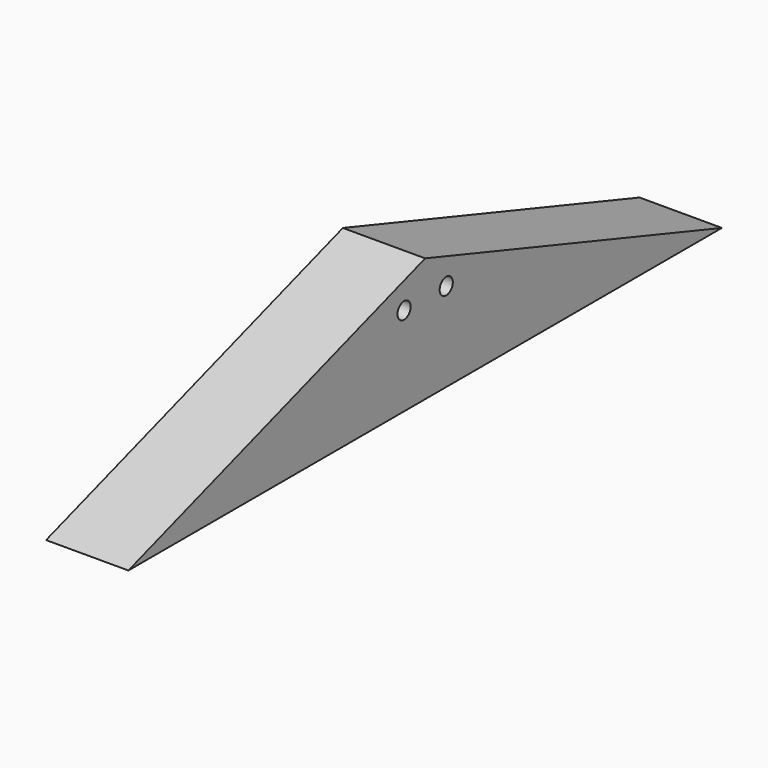
from build123d import *

# Parameters (mm, degrees)
F1_DEPTH  = 8
F3_DEPTH  = 621.7
F4_DEPTH  = 5.5
F7_DEPTH  = 5.5
F9_DEPTH  = 5.5
F11_DEPTH = 5.5
F13_DEPTH = 5.5
F15_DEPTH = 5.5
F17_DEPTH = 308.2
F18_DEPTH = 24
F20_DEPTH = 244.2
F21_DEPTH = 30.35
F22_R     = 2.5
F23_DEPTH = 0.5
F24_R     = 2.5
F25_DEPTH = 0.5
F26_R     = 2.5
F27_DEPTH = 0.5
F28_R     = 2.5
F29_DEPTH = 0.5
F30_W     = 14.1428571429
F30_H     = 18
F30_W_2   = 4.1785714286
F30_H_2   = 6.1071428571
F31_DEPTH = 0.5
F32_DEPTH = 25
F34_DEPTH = 8


# Not quite as in the source:
# - a feature of the source that left no trace in its solid (it failed there, or was rolled back) is left out


with BuildPart() as f1:
    # F0 (on Top) → F1 (new body)
    with BuildSketch(Plane.XY):
        Polygon((-327.3, 108.1424002851), (-327.3, -140.8575997149), (-102.6, -140.8575997149), (-102.6, -170.8575997149), (0, -170.8575997149), (0, -140.8575997149), (288.9, -140.8575997149), (288.9, 108.1424002851), (0, 108.1424002851), (0, 138.1424002851), (-102.6, 128.6424002851), (-102.6, 108.1424002851), align=None)
    extrude(amount=F1_DEPTH)

    # F2 (on face) → F3 (join)
    with BuildSketch(Plane.YZ.offset(288.9)):
        Polygon((-16.3575997149, 51.4532495908), (-146.3575997149, 8), (-140.8575997149, 8), (108.1424002851, 8), (113.6424002851, 8), align=None)
    extrude(amount=-F3_DEPTH)

    # F2 (on face) → F4 (join)
    with BuildSketch(Plane.YZ.offset(288.9)):
        Polygon((-16.3575997149, 51.4532495908), (-146.3575997149, 8), (113.6424002851, 8), align=None)
    extrude(amount=F4_DEPTH)

    # F5 (on face) → F7 (join)
    with BuildSketch(Plane.XZ.offset(170.8575997149)):
        Polygon((-51.3, 62.75), (-108.1, 8), (5.5, 8), align=None)
    extrude(amount=F7_DEPTH)

    # F8 (on face) → F9 (cut)
    with BuildSketch(Plane(origin=(-13.187163576, 142.4213666207, 0), x_dir=(-0.9957406741, -0.0921982106, 0), z_dir=(-0.0921982106, 0.9957406741, 0))):
        Polygon((91.8565413643, 4.3927081219), (38.2758658123, 55.8195932448), (-15.3048097397, 4.3927081219), align=None)
    extrude(amount=-F9_DEPTH, mode=Mode.SUBTRACT)

    # F10 (on face) → F11 (cut)
    with BuildSketch(Plane(origin=(-332.8, 0, 0), x_dir=(0, -1, 0), z_dir=(-1, 0, 0))):
        Polygon((144.6140170728, 2.7836871671), (16.3575997149, 45.6541342062), (-111.8988176431, 2.7836871671), align=None)
    extrude(amount=-F11_DEPTH, mode=Mode.SUBTRACT)

    # F12 (on face) → F13 (cut)
    with BuildSketch(Plane.YZ.offset(294.4)):
        Polygon((111.8988176431, 2.7836871671), (-16.3575997149, 45.6541342062), (-144.6140170728, 2.7836871671), align=None)
    extrude(amount=-F13_DEPTH, mode=Mode.SUBTRACT)

    # F14 (on face) → F15 (cut)
    with BuildSketch(Plane.XZ.offset(176.3575997149)):
        Polygon((1.6830285492, 4.0401099834), (-51.3, 55.1108989459), (-104.2830285492, 4.0401099834), align=None)
    extrude(amount=-F15_DEPTH, mode=Mode.SUBTRACT)

    # F16 (on face) → F17 (join)
    with BuildSketch(Plane.YZ.offset(294.4)):
        Polygon((-37.9123742622, 48.4659791319), (-36.6443145321, 44.6722981882), (-16.3575997149, 51.4532495908), (3.9291151024, 44.6722981882), (5.1971748325, 48.4659791319), (-16.3575997149, 55.670786811), align=None)
    extrude(amount=-F17_DEPTH)

    # F16 (on face) → F18 (cut)
    with BuildSketch(Plane.YZ.offset(294.4)):
        Polygon((-37.9123742622, 48.4659791319), (-36.6443145321, 44.6722981882), (-16.3575997149, 51.4532495908), (3.9291151024, 44.6722981882), (5.1971748325, 48.4659791319), (-16.3575997149, 55.670786811), align=None)
    extrude(amount=-F18_DEPTH, mode=Mode.SUBTRACT)

    # F19 (on face) → F20 (join)
    with BuildSketch(Plane(origin=(-332.8, 0, 0), x_dir=(0, -1, 0), z_dir=(-1, 0, 0))):
        Polygon((-5.1971748325, 48.4659791319), (-3.9291151024, 44.6722981882), (16.3575997149, 51.4532495908), (36.6443145321, 44.6722981882), (37.9123742622, 48.4659791319), (16.3575997149, 55.670786811), align=None)
    extrude(amount=-F20_DEPTH)

    # F19 (on face) → F21 (cut)
    with BuildSketch(Plane(origin=(-332.8, 0, 0), x_dir=(0, -1, 0), z_dir=(-1, 0, 0))):
        Polygon((-5.1971748325, 48.4659791319), (-3.9291151024, 44.6722981882), (16.3575997149, 51.4532495908), (36.6443145321, 44.6722981882), (37.9123742622, 48.4659791319), (16.3575997149, 55.670786811), align=None)
    extrude(amount=-F21_DEPTH, mode=Mode.SUBTRACT)

    # F22 (on face) → F23 (cut)
    with BuildSketch(Plane(origin=(-327.3, 0, 0), x_dir=(0, -1, 0), z_dir=(-1, 0, 0))):
        with Locations((8.3575997149, 35)):
            Circle(F22_R)
        with Locations((24.3575997149, 35)):
            Circle(F22_R)
    extrude(amount=-F23_DEPTH, mode=Mode.SUBTRACT)

    # F24 (on face) → F25 (cut)
    with BuildSketch(Plane.YZ.offset(288.9)):
        with Locations((-24.3575997149, 35)):
            Circle(F24_R)
        with Locations((-8.3575997149, 35)):
            Circle(F24_R)
    extrude(amount=-F25_DEPTH, mode=Mode.SUBTRACT)

    # F26 (on face) → F27 (cut)
    with BuildSketch(Plane.XZ.offset(170.8575997149)):
        with Locations((-59.3, 35)):
            Circle(F26_R)
        with Locations((-43.3, 35)):
            Circle(F26_R)
    extrude(amount=-F27_DEPTH, mode=Mode.SUBTRACT)

    # F28 (on face) → F29 (cut)
    with BuildSketch(Plane(origin=(-12.6822332802, 136.9681194259, 0), x_dir=(-0.9957406741, -0.0921982106, 0), z_dir=(-0.0921982106, 0.9957406741, 0))):
        with Locations((30.7829559704, 35)):
            Circle(F28_R)
        with Locations((46.7829559704, 35)):
            Circle(F28_R)
    extrude(amount=-F29_DEPTH, mode=Mode.SUBTRACT)

    # F30 (on face) → F31 (cut)
    with BuildSketch(Plane.YZ.offset(288.9)):
        with Locations((-16.3575997149, 14)):
            Rectangle(F30_W, F30_H)
        with Locations((-19.4111711434, 9.9821428571)):
            Rectangle(F30_W_2, F30_H_2, mode=Mode.SUBTRACT)
        with Locations((-13.3040282863, 9.9821428571)):
            Rectangle(F30_W_2, F30_H_2, mode=Mode.SUBTRACT)
        with Locations((-19.4111711434, 18.0178571429)):
            Rectangle(F30_W_2, F30_H_2, mode=Mode.SUBTRACT)
        with Locations((-13.3040282863, 18.0178571429)):
            Rectangle(F30_W_2, F30_H_2, mode=Mode.SUBTRACT)
        with Locations((18.6424002851, 14)):
            Rectangle(F30_W, F30_H)
        with Locations((15.5888288566, 9.9821428571)):
            Rectangle(F30_W_2, F30_H_2, mode=Mode.SUBTRACT)
        with Locations((21.6959717137, 9.9821428571)):
            Rectangle(F30_W_2, F30_H_2, mode=Mode.SUBTRACT)
        with Locations((15.5888288566, 18.0178571429)):
            Rectangle(F30_W_2, F30_H_2, mode=Mode.SUBTRACT)
        with Locations((21.6959717137, 18.0178571429)):
            Rectangle(F30_W_2, F30_H_2, mode=Mode.SUBTRACT)
        with Locations((-51.3575997149, 14)):
            Rectangle(F30_W, F30_H)
        with Locations((-54.4111711434, 9.9821428571)):
            Rectangle(F30_W_2, F30_H_2, mode=Mode.SUBTRACT)
        with Locations((-48.3040282863, 9.9821428571)):
            Rectangle(F30_W_2, F30_H_2, mode=Mode.SUBTRACT)
        with Locations((-54.4111711434, 18.0178571429)):
            Rectangle(F30_W_2, F30_H_2, mode=Mode.SUBTRACT)
        with Locations((-48.3040282863, 18.0178571429)):
            Rectangle(F30_W_2, F30_H_2, mode=Mode.SUBTRACT)
    extrude(amount=-F31_DEPTH, mode=Mode.SUBTRACT)


with BuildPart() as f32:
    # F32 (new): a face of the model
    f32_faces = [f1.part.faces().sort_by_distance(p)[0] for p in [
        (-327.3, -16.3575997149, 15.1372563079),
    ]]
    extrude(f32_faces, amount=F32_DEPTH)

    # F34 (cut): a face of the model
    f34_faces = [f32.faces().sort_by_distance(p)[0] for p in [
        (-339.8, -16.3575997149, 0),
    ]]
    extrude(f34_faces, amount=-F34_DEPTH, mode=Mode.SUBTRACT)


solid = f32.part
